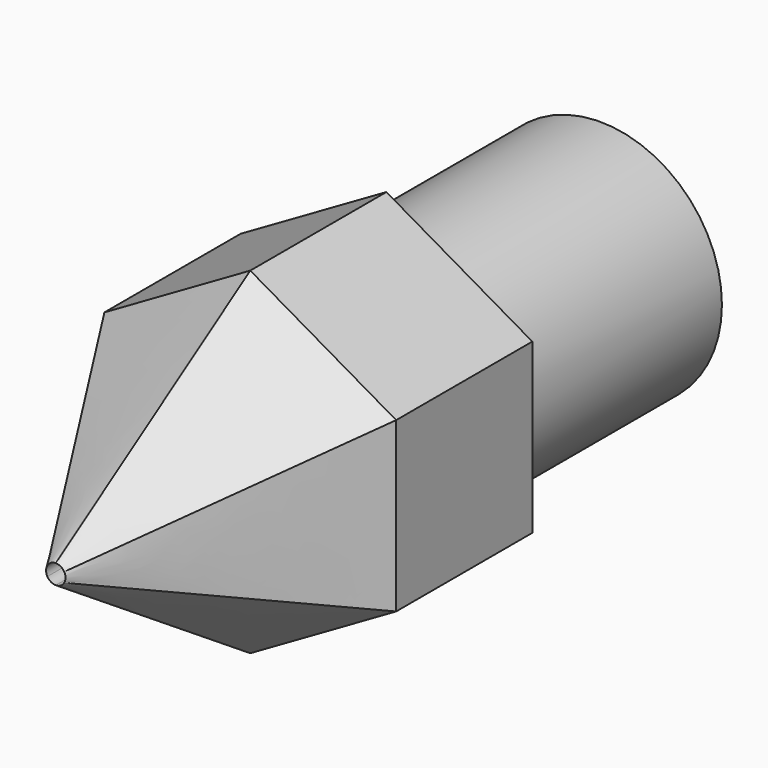
from build123d import *

# Parameters (mm, degrees)
F0_R     = 2.5
F1_DEPTH = 5.5
F2_R     = 2.5
F3_DEPTH = 3.5
F7_DEPTH = 25


# Not quite as in the source:
# - the arcs of a loft's sections are written as splines that run evenly, so that the points pair up as in the source's solid


with BuildPart() as f1:
    # F0 (on Front) → F1 (new body)
    with BuildSketch(Plane.XZ):
        Circle(F0_R)
    extrude(amount=F1_DEPTH)

    # F2 (on face) → F3 (join)
    with BuildSketch(Plane.XZ.offset(5.5)):
        Polygon((3, -1.7320508076), (3, 1.7320508076), (0, 3.4641016151), (-3, 1.7320508076), (-3, -1.7320508076), (0, -3.4641016151), align=None)
        Circle(F2_R, mode=Mode.SUBTRACT)
        Circle(F2_R)
    extrude(amount=F3_DEPTH)

    # F5 (on offset) → F6 section 0
    with BuildSketch(Plane.XZ.offset(14)):
        with BuildLine():
            add(Edge.make_bspline(
                [(0.1732050808, -0.1), (0.1848406091, -0.0798466737), (0.192920574, -0.0576471526), (0.2010025272, -0.0118121185), (0.2010025272, 0.0118121185), (0.192920574, 0.0576471526), (0.1848406091, 0.0798466737), (0.1732050808, 0.1)],
                knots=[0, 0, 0, 0, 0.3333333333, 0.3333333333, 0.6666666667, 0.6666666667, 1, 1, 1, 1], degree=3))
            add(Edge.make_bspline(
                [(0.1732050808, 0.1), (0.1615695524, 0.1201533263), (0.1463841856, 0.1382505417), (0.1107308583, 0.1681672355), (0.0902716689, 0.179979354), (0.0465363884, 0.1958976943), (0.0232710567, 0.2), (0, 0.2)],
                knots=[0, 0, 0, 0, 0.3333333333, 0.3333333333, 0.6666666667, 0.6666666667, 1, 1, 1, 1], degree=3))
            add(Edge.make_bspline(
                [(0, 0.2), (-0.0232710567, 0.2), (-0.0465363884, 0.1958976943), (-0.0902716689, 0.179979354), (-0.1107308583, 0.1681672355), (-0.1463841856, 0.1382505417), (-0.1615695524, 0.1201533263), (-0.1732050808, 0.1)],
                knots=[0, 0, 0, 0, 0.3333333333, 0.3333333333, 0.6666666667, 0.6666666667, 1, 1, 1, 1], degree=3))
            add(Edge.make_bspline(
                [(-0.1732050808, 0.1), (-0.1848406091, 0.0798466737), (-0.192920574, 0.0576471526), (-0.2010025272, 0.0118121185), (-0.2010025272, -0.0118121185), (-0.192920574, -0.0576471526), (-0.1848406091, -0.0798466737), (-0.1732050808, -0.1)],
                knots=[0, 0, 0, 0, 0.3333333333, 0.3333333333, 0.6666666667, 0.6666666667, 1, 1, 1, 1], degree=3))
            add(Edge.make_bspline(
                [(-0.1732050808, -0.1), (-0.1615695524, -0.1201533263), (-0.1463841856, -0.1382505417), (-0.1107308583, -0.1681672355), (-0.0902716689, -0.179979354), (-0.0465363884, -0.1958976943), (-0.0232710567, -0.2), (0, -0.2)],
                knots=[0, 0, 0, 0, 0.3333333333, 0.3333333333, 0.6666666667, 0.6666666667, 1, 1, 1, 1], degree=3))
            add(Edge.make_bspline(
                [(0, -0.2), (0.0232710567, -0.2), (0.0465363884, -0.1958976943), (0.0902716689, -0.179979354), (0.1107308583, -0.1681672355), (0.1463841856, -0.1382505417), (0.1615695524, -0.1201533263), (0.1732050808, -0.1)],
                knots=[0, 0, 0, 0, 0.3333333333, 0.3333333333, 0.6666666667, 0.6666666667, 1, 1, 1, 1], degree=3))
        make_face()
    # F3_face (on face) → F6 section 1
    with BuildSketch(Plane.XZ.offset(9)):
        Polygon((3, -1.7320508076), (3, 1.7320508076), (0, 3.4641016151), (-3, 1.7320508076), (-3, -1.7320508076), (0, -3.4641016151), align=None)
    loft(ruled=True)

    # F7 (cut): a face of the model
    f7_faces = [f1.faces().sort_by_distance(p)[0] for p in [
        (0, -14, 0),
    ]]
    extrude(f7_faces, amount=-F7_DEPTH, mode=Mode.SUBTRACT)


solid = f1.part
